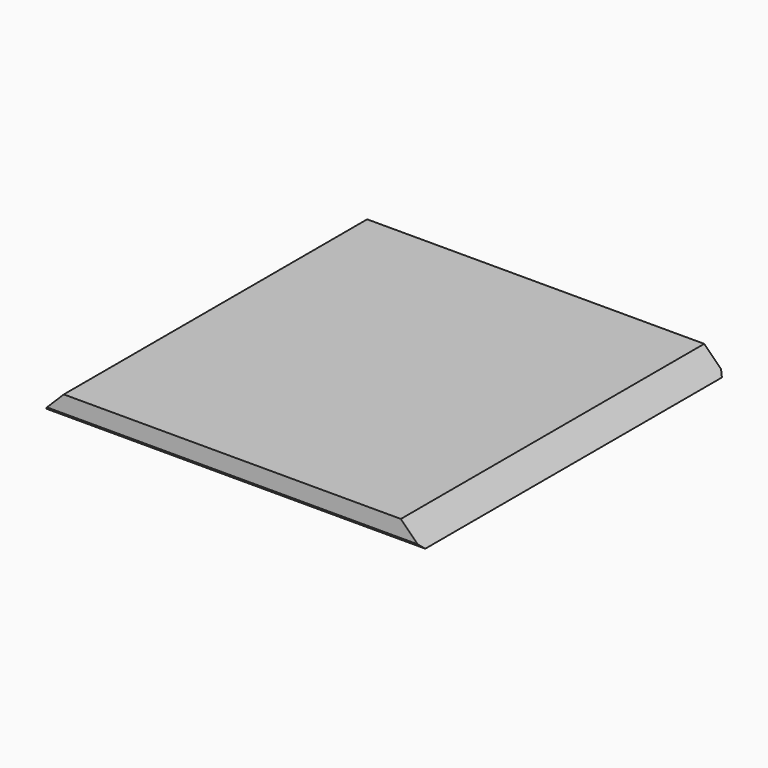
from build123d import *

# Parameters (mm, degrees)
F0_W     = 450
F0_H     = 25
F1_DEPTH = 450
F2_SIZE  = 24.99999
F3_SIZE  = 24.99999
F4_SIZE  = 5


# Not quite as in the source:
# - a fillet or chamfer is up to 0.001 mm smaller than in the source, because OpenCascade refuses the exact size


with BuildPart() as f1:
    # F0 (on Front) → F1 (new body)
    with BuildSketch(Plane.XZ):
        with Locations((269.2221287504, -20.1100035338)):
            Rectangle(F0_W, F0_H)
    extrude(amount=F1_DEPTH)

    # F2 (size 25 in the source; OpenCascade refuses exactly that, so slightly less here)
    f2_edges = [f1.edges().sort_by_distance(p)[0] for p in [
        (44.222129, -225, -7.610004),
    ]]
    chamfer(f2_edges, length=F2_SIZE)

    # F3 (size 25 in the source; OpenCascade refuses exactly that, so slightly less here)
    f3_edges = [f1.edges().sort_by_distance(p)[0] for p in [
        (494.222129, -225, -7.610004),
    ]]
    chamfer(f3_edges, length=F3_SIZE)

    # F4
    f4_edges = [f1.edges().sort_by_distance(p)[0] for p in [
        (269.222129, -450, -32.610004),
        (269.222129, 0, -32.610004),
    ]]
    chamfer(f4_edges, length=F4_SIZE)


solid = f1.part
